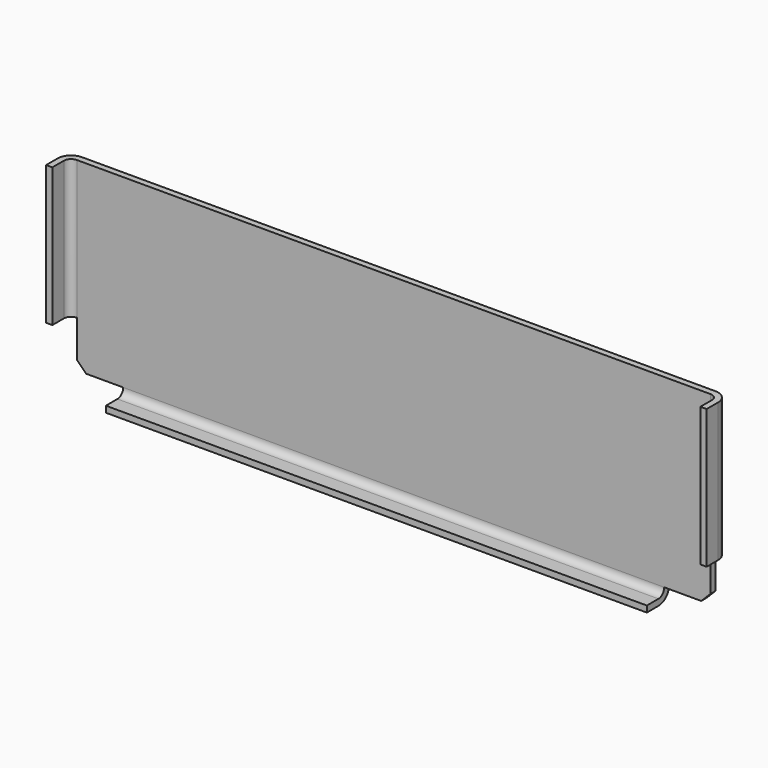
from build123d import *

# Parameters (mm, degrees)
F1_DEPTH = 101.6
F2_W     = 347.66504
F2_H     = 7.38632
F3_DEPTH = 3.41884
F4_W     = 347.66504
F4_H     = 3.41884
F5_DEPTH = 11.90498
F6_R     = 3.96748
F7_R     = 7.38632
F8_W     = 7.38632
F8_H     = 25.4
F8_W_2   = 25.4
F8_H_2   = 7.38632
F9_DEPTH = 15.32382
F10_SIZE = 5.08


# Not quite as in the source:
# - a feature names something its author has since deleted; it is built from what else it names


with BuildPart() as f1:
    # F0 (on Top) → F1 (new body)
    with BuildSketch(Plane.XY):
        Polygon((-3.41884, 0), (0, 0), (0, 11.90498), (355.6, 11.90498), (355.6, 0), (359.01884, 0), (359.01884, 15.32382), (-3.41884, 15.32382), align=None)
    extrude(amount=F1_DEPTH)

    # F2 (on face) → F3 (join, through all)
    with BuildSketch(Plane(origin=(0, 15.32382, 0), x_dir=(-1, 0, 0), z_dir=(0, 1, 0))):
        with Locations((-177.8, -3.69316)):
            Rectangle(F2_W, F2_H)
    extrude(amount=-F3_DEPTH)

    # F4 (on face) → F5 (join, through all)
    with BuildSketch(Plane.XZ.offset(-11.90498)):
        with Locations((177.8, -5.6769)):
            Rectangle(F4_W, F4_H)
    extrude(amount=F5_DEPTH)

    # F6
    f6_edges = [f1.edges().sort_by_distance(p)[0] for p in [
        (0, 11.90498, 50.8),
        (355.6, 11.90498, 50.8),
        (177.8, 11.90498, -3.96748),
    ]]
    fillet(f6_edges, radius=F6_R)

    # F7
    f7_edges = [f1.edges().sort_by_distance(p)[0] for p in [
        (-3.41884, 15.32382, 50.8),
        (359.01884, 15.32382, 50.8),
        (177.8, 15.32382, -7.38632),
    ]]
    fillet(f7_edges, radius=F7_R)

    # F8 (on face) → F9 (cut, through all)
    with BuildSketch(Plane(origin=(0, 15.32382, 0), x_dir=(-1, 0, 0), z_dir=(0, 1, 0))):
        with Locations((-355.32568, 12.7)):
            Rectangle(F8_W, F8_H)
        with Locations((-338.93252, -3.69316)):
            Rectangle(F8_W_2, F8_H_2)
        with Locations((-0.27432, 12.7)):
            Rectangle(F8_W, F8_H)
        with Locations((-16.66748, -3.69316)):
            Rectangle(F8_W_2, F8_H_2)
    extrude(amount=-F9_DEPTH, mode=Mode.SUBTRACT)

    # F10
    f10_edges = [f1.edges().sort_by_distance(p)[0] for p in [
        (351.63252, 13.6144, 0),
        (3.96748, 13.6144, 0),
    ]]
    chamfer(f10_edges, length=F10_SIZE)


solid = f1.part
